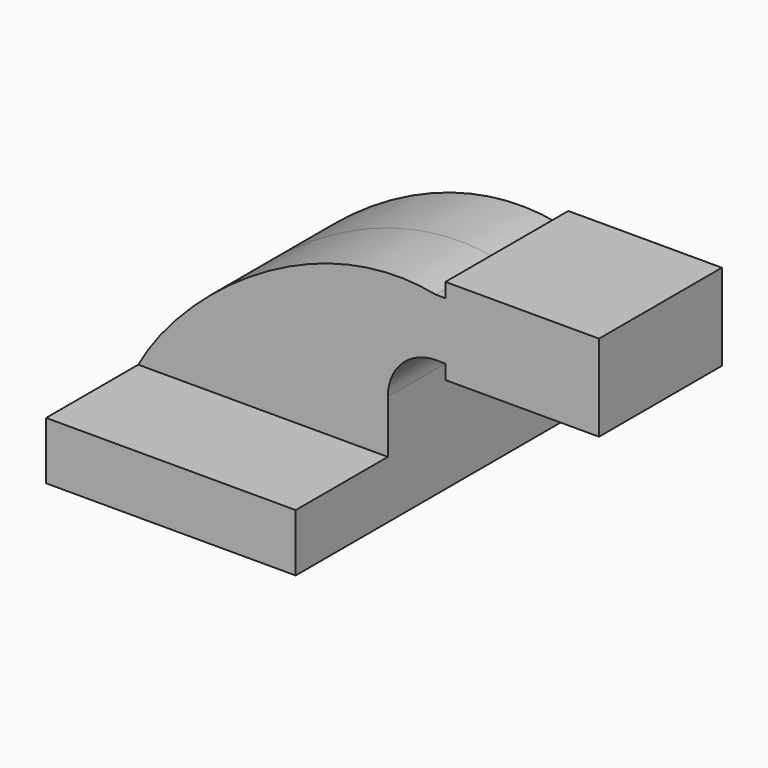
from build123d import *

# Parameters (mm, degrees)
F1_DEPTH = 63.5
F0_W     = 25.4
F0_H     = 19.05
F0_H_2   = 4.7498
F0_H_3   = 4.7752
F2_DEPTH = 25.4


with BuildPart() as f1:
    # F0 (on Front) → F1 (new body, symmetric)
    with BuildSketch(Plane.XZ):
        Polygon((-41.275, 9.525), (-41.275, -9.525), (41.275, -9.525), (41.275, 9.525), (22.225, 9.525), align=None)
    extrude(amount=F1_DEPTH, both=True)

    # F0 (on Front) → F2 (join, symmetric)
    with BuildSketch(Plane.XZ):
        Polygon((-41.275, 9.525), (-41.275, -9.525), (41.275, -9.525), (41.275, 9.525), (22.225, 9.525), align=None)
        with BuildLine():
            add(Edge.make_bspline(
                [(-41.275, 9.525), (-26.6867671162, 36.4819094539), (17.2914229333, 70.0652599335), (57.15, 61.9252)],
                knots=[0, 0, 0, 0, 111.5045361635, 111.5045361635, 111.5045361635, 111.5045361635], degree=3))
            Line((-41.275, 9.525), (22.225, 9.525))
            Line((22.225, 9.525), (22.225, 27.0002))
            ThreePointArc((22.225, 27.0002), (32.4542956671, 51.6959043329), (57.15, 61.9252))
        make_face()
        with BuildLine():
            Line((22.225, 9.525), (41.275, 9.525))
            Line((41.275, 9.525), (41.275, 27.0002))
            ThreePointArc((41.275, 27.0002), (45.9246798487, 38.2255201513), (57.15, 42.8752))
            Line((57.15, 42.8752), (60.325, 42.8752))
            Line((60.325, 42.8752), (60.325, 61.9252))
            Line((60.325, 61.9252), (57.15, 61.9252))
            ThreePointArc((57.15, 61.9252), (32.4542956671, 51.6959043329), (22.225, 27.0002))
            Line((22.225, 27.0002), (22.225, 9.525))
        make_face()
        with Locations((73.025, 52.4002)):
            Rectangle(F0_W, F0_H)
        with Locations((73.025, 64.3001)):
            Rectangle(F0_W, F0_H_2)
        with Locations((73.025, 40.4876)):
            Rectangle(F0_W, F0_H_3)
        Polygon((85.725, 66.675), (85.725, 61.9252), (85.725, 42.8752), (85.725, 38.1), (111.125, 38.1), (111.125, 66.675), align=None)
    extrude(amount=F2_DEPTH, both=True)


solid = f1.part
